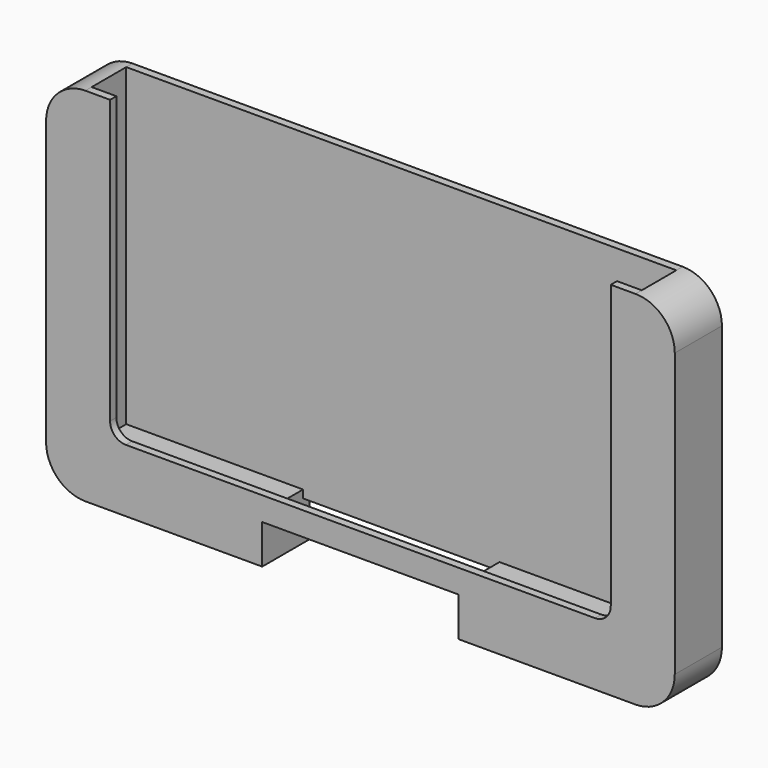
from build123d import *

# Parameters (mm, degrees)
F0_W     = 203.2
F0_H     = 116.84
F1_DEPTH = 19.05
F2_W     = 177.8
F2_H     = 13.97
F3_DEPTH = 101.6
F4_W     = 161.8175851255
F4_H     = 96.52
F5_DEPTH = 2.54
F6_W     = 63.5
F6_H     = 13.97
F7_DEPTH = 15.241
F8_W     = 63.5
F8_H     = 12.7
F9_DEPTH = 19.051
F10_R    = 12.69999
F11_R    = 5.08


# Not quite as in the source:
# - a fillet or chamfer is up to 0.001 mm smaller than in the source, because OpenCascade refuses the exact size


with BuildPart() as f1:
    # F0 (on Front) → F1 (new body)
    with BuildSketch(Plane.XZ):
        with Locations((101.6, 58.42)):
            Rectangle(F0_W, F0_H)
    extrude(amount=F1_DEPTH)

    # F2 (on face) → F3 (cut)
    with BuildSketch(Plane.XY.offset(116.84)):
        with Locations((101.6, -9.525)):
            Rectangle(F2_W, F2_H)
    extrude(amount=-F3_DEPTH, mode=Mode.SUBTRACT)

    # F4 (on face) → F5 (cut, through all)
    with BuildSketch(Plane.XZ.offset(19.05)):
        with Locations((101.6, 68.58)):
            Rectangle(F4_W, F4_H)
    extrude(amount=-F5_DEPTH, mode=Mode.SUBTRACT)

    # F6 (on face) → F7 (cut, through all)
    with BuildSketch(Plane.XY.offset(15.24)):
        with Locations((101.6, -9.525)):
            Rectangle(F6_W, F6_H)
    extrude(amount=-F7_DEPTH, mode=Mode.SUBTRACT)

    # F8 (on face) → F9 (cut, through all)
    with BuildSketch(Plane.XZ.offset(19.05)):
        with Locations((101.6, 6.35)):
            Rectangle(F8_W, F8_H)
    extrude(amount=-F9_DEPTH, mode=Mode.SUBTRACT)

    # F10 (radius 12.7 in the source; OpenCascade refuses exactly that, so slightly less here)
    f10_edges = [f1.edges().sort_by_distance(p)[0] for p in [
        (0, -9.525, 116.84),
        (0, -9.525, 0),
        (203.2, -9.525, 0),
        (203.2, -9.525, 116.84),
    ]]
    fillet(f10_edges, radius=F10_R)

    # F11
    f11_edges = [f1.edges().sort_by_distance(p)[0] for p in [
        (20.691207, -17.78, 20.32),
        (182.508793, -17.78, 20.32),
    ]]
    fillet(f11_edges, radius=F11_R)


solid = f1.part
